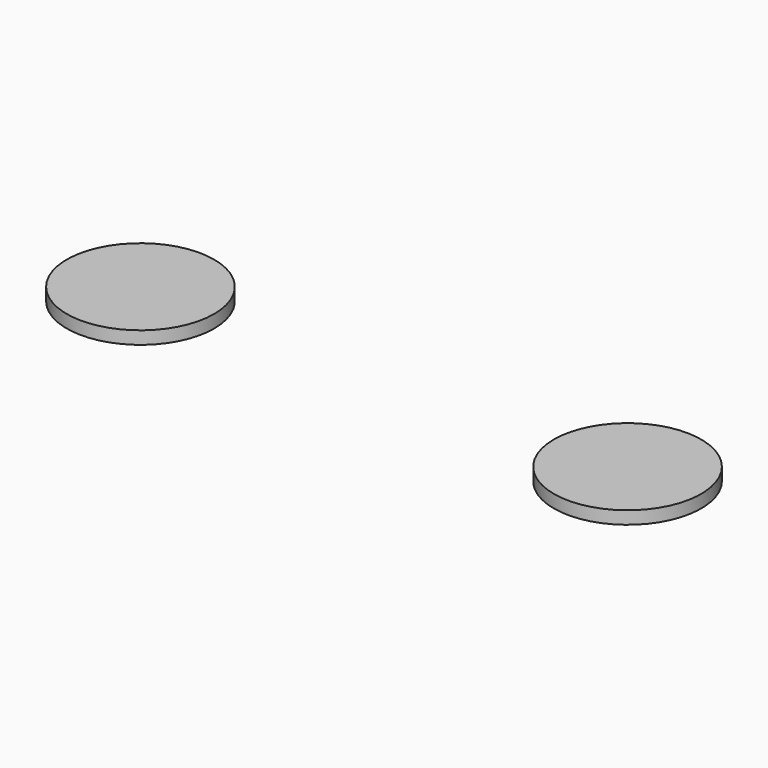
from build123d import *

# Parameters (mm, degrees)
F1_DEPTH = 2
F0_R     = 11.5
F0_R_2   = 4


# Not quite as in the source:
# - the program builds the solid bodies; features that only make, move or delete a surface that nothing else refers to are left out


with BuildPart() as f1:
    # F0 (on Top) → F1 (new body)
    with BuildSketch(Plane.XY):
        with BuildLine():
            ThreePointArc((49.5, 0), (38, 11.5), (26.5, 0))
            ThreePointArc((26.5, 0), (38, -11.5), (49.5, 0))
        make_face()
        with BuildLine():
            ThreePointArc((42, 0), (38, -4), (34, 0))
            ThreePointArc((34, 0), (38, 4), (42, 0))
        make_face(mode=Mode.SUBTRACT)
        with BuildLine():
            ThreePointArc((42, 0), (38, 4), (34, 0))
            ThreePointArc((34, 0), (38, -4), (42, 0))
        make_face()
    extrude(amount=F1_DEPTH)


with BuildPart() as f1b:
    # F0 (on Top) → F1, piece 2 (new body)
    with BuildSketch(Plane.XY):
        with Locations((-38, 0)):
            Circle(F0_R)
        with Locations((-38, 0)):
            Circle(F0_R_2, mode=Mode.SUBTRACT)
        with Locations((-38, 0)):
            Circle(F0_R_2)
    extrude(amount=F1_DEPTH)


solid = Compound([f1.part, f1b.part])
